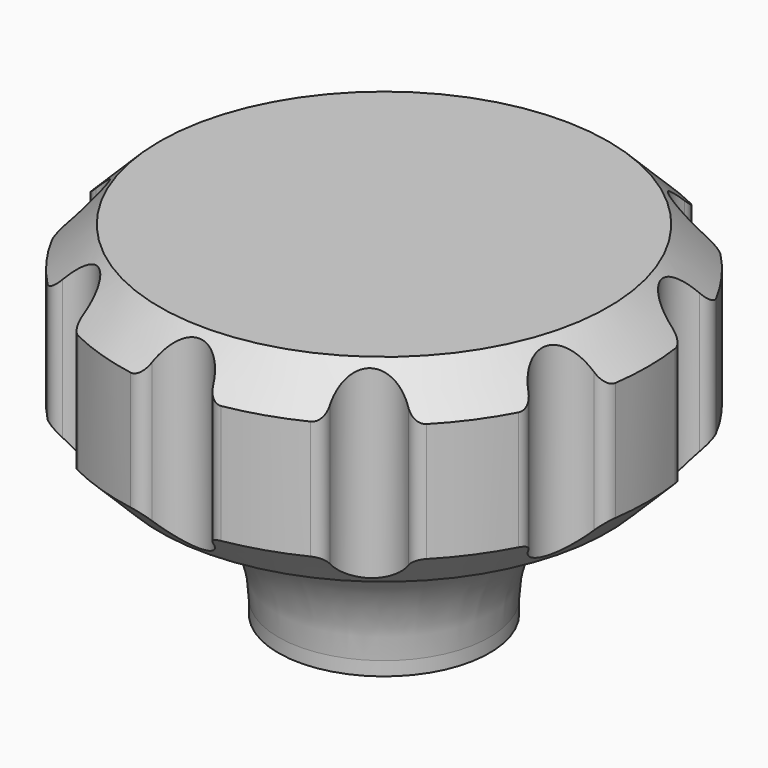
from build123d import *

# Parameters (mm, degrees)
F3_SIZE     = 3
F2_R        = 2.5
F4_DEPTH    = 25
F5_T1_DEPTH = 13.7188854723
F7_R        = 1.9
F8_DEPTH    = 25


# Not quite as in the source:
# - a fillet or chamfer that OpenCascade refuses, or shapes differently, is made with other operations: its cross-section is extruded or revolved along the edge and cut away or added


with BuildPart() as f1:
    # F0 (on Front) → F1 (revolve)
    with BuildSketch(Plane.XZ):
        Polygon((-4.1, 8), (0, 8), (0, 26), (-20, 26), (-20, 11), (-8, 11), (-8, 0), (-4.1, 0), align=None)
    revolve(axis=Axis((0, 0, 3.9634779096), (0, 0, -1)))

    # F3
    f3_edges = [f1.edges().sort_by_distance(p)[0] for p in [
        (20, 0, 26),
        (20, 0, 11),
    ]]
    chamfer(f3_edges, length=F3_SIZE)

    # F2 (on face) → F4 (cut)
    with BuildSketch(Plane.XY.offset(26)):
        with Locations((0, 20)):
            Circle(F2_R)
        with Locations((-11.7557050458, 16.1803398875)):
            Circle(F2_R)
        with Locations((-19.0211303259, 6.1803398875)):
            Circle(F2_R)
        with Locations((-19.0211303259, -6.1803398875)):
            Circle(F2_R)
        with Locations((-11.7557050458, -16.1803398875)):
            Circle(F2_R)
        with Locations((0, -20)):
            Circle(F2_R)
        with Locations((11.7557050458, -16.1803398875)):
            Circle(F2_R)
        with Locations((19.0211303259, -6.1803398875)):
            Circle(F2_R)
        with Locations((19.0211303259, 6.1803398875)):
            Circle(F2_R)
        with Locations((11.7557050458, 16.1803398875)):
            Circle(F2_R)
    extrude(amount=-F4_DEPTH, mode=Mode.SUBTRACT)

    # F5: fillet of radius 1 on 20 edges, made by hand

    # F5_s2 → F5_t1 (cut)
    with BuildSketch(Plane.XY.offset(11.6405572638)):
        with BuildLine():
            ThreePointArc((-8.8079930969, -17.9560368012), (-9.276305167, -17.4756592069), (-9.3356253289, -16.8074077972))
            ThreePointArc((-9.3356253289, -16.8074077972), (-9.4625605244, -17.1760748942), (-9.6452752578, -17.5205212594))
            ThreePointArc((-9.6452752578, -17.5205212594), (-9.2292034699, -17.7432185161), (-8.8079930969, -17.9560368012))
        make_face()
        with BuildLine():
            ThreePointArc((-13.0999278278, -14.0724819434), (-13.7538036236, -14.222566159), (-14.3553862533, -13.9256197535))
            ThreePointArc((-14.3553862533, -13.9256197535), (-14.0228228731, -14.2604501567), (-13.6824519426, -14.5873407048))
            ThreePointArc((-13.6824519426, -14.5873407048), (-13.4113259402, -14.3071288865), (-13.0999278278, -14.0724819434))
        make_face()
        with BuildLine():
            ThreePointArc((-17.6801097231, -9.3495304791), (-17.776623281, -8.6856299133), (-17.4318259766, -8.1101356501))
            ThreePointArc((-17.4318259766, -8.1101356501), (-17.7512157896, -8.3337829609), (-18.1014956077, -8.5050488983))
            ThreePointArc((-18.1014956077, -8.5050488983), (-17.8957846237, -8.9297756244), (-17.6801097231, -9.3495304791))
        make_face()
        with BuildLine():
            ThreePointArc((-18.8696615873, -3.684932662), (-19.4868755069, -3.4220147934), (-19.7990253599, -2.8281787071))
            ThreePointArc((-19.7990253599, -2.8281787071), (-19.7267843066, -3.2945380439), (-19.6435598827, -3.7590630659))
            ThreePointArc((-19.6435598827, -3.7590630659), (-19.2595099649, -3.6917308086), (-18.8696615873, -3.684932662))
        make_face()
        with BuildLine():
            ThreePointArc((-17.4318259766, 8.1101356501), (-17.776623281, 8.6856299133), (-17.6801097231, 9.3495304791))
            ThreePointArc((-17.6801097231, 9.3495304791), (-17.8957846237, 8.9297756244), (-18.1014956077, 8.5050488983))
            ThreePointArc((-18.1014956077, 8.5050488983), (-17.7512157896, 8.3337829609), (-17.4318259766, 8.1101356501))
        make_face()
        with BuildLine():
            ThreePointArc((-18.8696615873, 3.684932662), (-19.4868755069, 3.4220147934), (-19.7990253599, 2.8281787071))
            ThreePointArc((-19.7990253599, 2.8281787071), (-19.7267843066, 3.2945380439), (-19.6435598827, 3.7590630659))
            ThreePointArc((-19.6435598827, 3.7590630659), (-19.2595099649, 3.6917308086), (-18.8696615873, 3.684932662))
        make_face()
        with BuildLine():
            ThreePointArc((-14.3553862533, 13.9256197535), (-13.7538036236, 14.222566159), (-13.0999278278, 14.0724819434))
            ThreePointArc((-13.0999278278, 14.0724819434), (-13.4113259402, 14.3071288865), (-13.6824519426, 14.5873407048))
            ThreePointArc((-13.6824519426, 14.5873407048), (-14.0228228731, 14.2604501567), (-14.3553862533, 13.9256197535))
        make_face()
        with BuildLine():
            ThreePointArc((-9.3356253289, 16.8074077972), (-9.276305167, 17.4756592069), (-8.8079930969, 17.9560368012))
            ThreePointArc((-8.8079930969, 17.9560368012), (-9.2292034699, 17.7432185161), (-9.6452752578, 17.5205212594))
            ThreePointArc((-9.6452752578, 17.5205212594), (-9.4625605244, 17.1760748942), (-9.3356253289, 16.8074077972))
        make_face()
        with BuildLine():
            ThreePointArc((-3.4284775196, 19.7039473684), (-2.7672462308, 19.5905806592), (-2.3264668883, 19.0848214286))
            ThreePointArc((-2.3264668883, 19.0848214286), (-2.4404712406, 19.4576900113), (-2.4951124098, 19.84375))
            ThreePointArc((-2.4951124098, 19.84375), (-2.9626197203, 19.7793550045), (-3.4284775196, 19.7039473684))
        make_face()
        with BuildLine():
            ThreePointArc((2.3264668883, 19.0848214286), (2.7672462308, 19.5905806592), (3.4284775196, 19.7039473684))
            ThreePointArc((3.4284775196, 19.7039473684), (2.9626197203, 19.7793550045), (2.4951124098, 19.84375))
            ThreePointArc((2.4951124098, 19.84375), (2.4404712406, 19.4576900113), (2.3264668883, 19.0848214286))
        make_face()
        with BuildLine():
            ThreePointArc((8.8079930969, 17.9560368012), (9.276305167, 17.4756592069), (9.3356253289, 16.8074077972))
            ThreePointArc((9.3356253289, 16.8074077972), (9.4625605244, 17.1760748942), (9.6452752578, 17.5205212594))
            ThreePointArc((9.6452752578, 17.5205212594), (9.2292034699, 17.7432185161), (8.8079930969, 17.9560368012))
        make_face()
        with BuildLine():
            ThreePointArc((13.0999278278, 14.0724819434), (13.7538036236, 14.222566159), (14.3553862533, 13.9256197535))
            ThreePointArc((14.3553862533, 13.9256197535), (14.0228228731, 14.2604501567), (13.6824519426, 14.5873407048))
            ThreePointArc((13.6824519426, 14.5873407048), (13.4113259402, 14.3071288865), (13.0999278278, 14.0724819434))
        make_face()
        with BuildLine():
            ThreePointArc((17.6801097231, 9.3495304791), (17.776623281, 8.6856299133), (17.4318259766, 8.1101356501))
            ThreePointArc((17.4318259766, 8.1101356501), (17.7512157896, 8.3337829609), (18.1014956077, 8.5050488983))
            ThreePointArc((18.1014956077, 8.5050488983), (17.8957846237, 8.9297756244), (17.6801097231, 9.3495304791))
        make_face()
        with BuildLine():
            ThreePointArc((18.8696615873, 3.684932662), (19.4868755069, 3.4220147934), (19.7990253599, 2.8281787071))
            ThreePointArc((19.7990253599, 2.8281787071), (19.7267843066, 3.2945380439), (19.6435598827, 3.7590630659))
            ThreePointArc((19.6435598827, 3.7590630659), (19.2595099649, 3.6917308086), (18.8696615873, 3.684932662))
        make_face()
        with BuildLine():
            ThreePointArc((19.7990253599, -2.8281787071), (19.4868755069, -3.4220147934), (18.8696615873, -3.684932662))
            ThreePointArc((18.8696615873, -3.684932662), (19.2595099649, -3.6917308086), (19.6435598827, -3.7590630659))
            ThreePointArc((19.6435598827, -3.7590630659), (19.7267843066, -3.2945380439), (19.7990253599, -2.8281787071))
        make_face()
        with BuildLine():
            ThreePointArc((17.4318259766, -8.1101356501), (17.776623281, -8.6856299133), (17.6801097231, -9.3495304791))
            ThreePointArc((17.6801097231, -9.3495304791), (17.8957846237, -8.9297756244), (18.1014956077, -8.5050488983))
            ThreePointArc((18.1014956077, -8.5050488983), (17.7512157896, -8.3337829609), (17.4318259766, -8.1101356501))
        make_face()
        with BuildLine():
            ThreePointArc((14.3553862533, -13.9256197535), (13.7538036236, -14.222566159), (13.0999278278, -14.0724819434))
            ThreePointArc((13.0999278278, -14.0724819434), (13.4113259402, -14.3071288865), (13.6824519426, -14.5873407048))
            ThreePointArc((13.6824519426, -14.5873407048), (14.0228228731, -14.2604501567), (14.3553862533, -13.9256197535))
        make_face()
        with BuildLine():
            ThreePointArc((9.3356253289, -16.8074077972), (9.276305167, -17.4756592069), (8.8079930969, -17.9560368012))
            ThreePointArc((8.8079930969, -17.9560368012), (9.2292034699, -17.7432185161), (9.6452752578, -17.5205212594))
            ThreePointArc((9.6452752578, -17.5205212594), (9.4625605244, -17.1760748942), (9.3356253289, -16.8074077972))
        make_face()
        with BuildLine():
            ThreePointArc((3.4284775196, -19.7039473684), (2.7672462308, -19.5905806592), (2.3264668883, -19.0848214286))
            ThreePointArc((2.3264668883, -19.0848214286), (2.4404712406, -19.4576900113), (2.4951124098, -19.84375))
            ThreePointArc((2.4951124098, -19.84375), (2.9626197203, -19.7793550045), (3.4284775196, -19.7039473684))
        make_face()
        with BuildLine():
            ThreePointArc((-2.3264668883, -19.0848214286), (-2.7672462308, -19.5905806592), (-3.4284775196, -19.7039473684))
            ThreePointArc((-3.4284775196, -19.7039473684), (-2.9626197203, -19.7793550045), (-2.4951124098, -19.84375))
            ThreePointArc((-2.4951124098, -19.84375), (-2.4404712406, -19.4576900113), (-2.3264668883, -19.0848214286))
        make_face()
    extrude(amount=F5_T1_DEPTH, mode=Mode.SUBTRACT)

    # F6: fillet of radius 10 on 1 edges, made by hand

    # F6_s1 → F6_t2 (revolve)
    with BuildSketch(Plane.XZ):
        with BuildLine():
            ThreePointArc((-17, 11), (-10.5838015129, 7.7583295614), (-8, 1.0501256289))
            Line((-8, 1.0501256289), (-7.8, 1.0501256289))
            Line((-7.8, 1.0501256289), (-7.8, 11))
            Line((-7.8, 11), (-8, 11.2))
            ThreePointArc((-8, 11.2), (-12.5, 11.2), (-16.98, 11.1989974874))
            Line((-16.98, 11.1989974874), (-17, 11))
        make_face()
    revolve(axis=Axis((0, 0, 11), (0, 0, -1)))

    # F7 (on Front) → F8 (cut)
    with BuildSketch(Plane.XZ):
        with Locations((0, 4.5)):
            Circle(F7_R)
    extrude(amount=-F8_DEPTH, mode=Mode.SUBTRACT)


solid = f1.part
